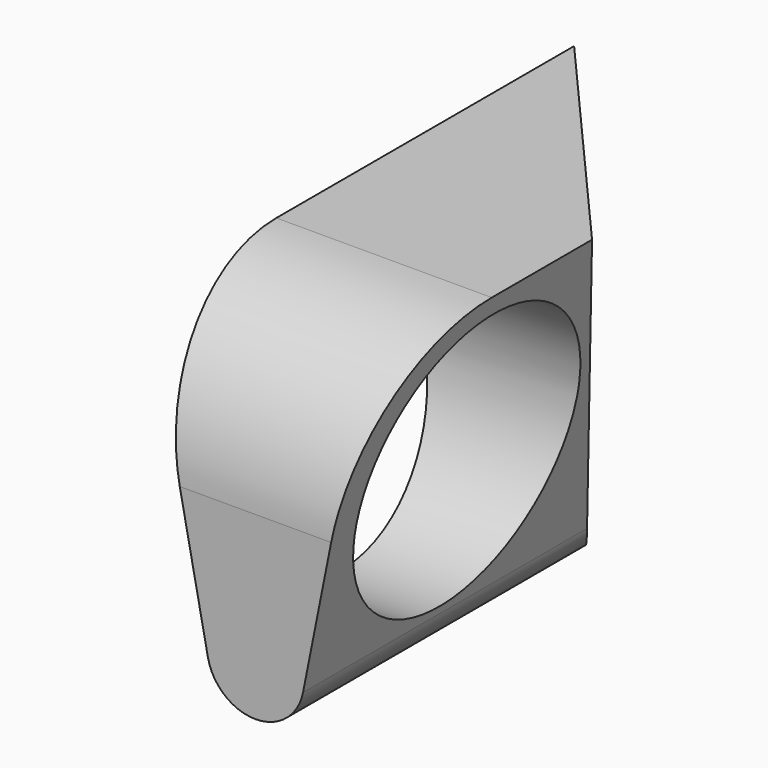
from build123d import *

# Parameters (mm, degrees)
F1_DEPTH      = 25
F2_T1_DEPTH   = 79.8532648187
F4_DEPTH      = 25
F4_DEPTH_BACK = 25
F5_T1_DEPTH   = 107.1220330496
F7_DEPTH      = 25
F8_R          = 6.2148490945
F9_DEPTH      = 25
F9_DEPTH_BACK = 25
F10_R         = 7.2426406871


# Not quite as in the source:
# - a fillet or chamfer that OpenCascade refuses, or shapes differently, is made with other operations: its cross-section is extruded or revolved along the edge and cut away or added


with BuildPart() as f1:
    # F0 (on Front) → F1 (new body)
    with BuildSketch(Plane.XZ):
        Polygon((4.8560337164, 7.4956272729), (0, 7.4956272729), (-4.8560337164, 7.4956272729), (0, -16.87037386), align=None)
    extrude(amount=F1_DEPTH)

    # F2: fillet of radius 2.1864014695 on 1 edges, made by hand

    # F2_s2 → F2_t1 (cut)
    with BuildSketch(Plane.XZ.offset(-27.4266324093)):
        with BuildLine():
            ThreePointArc((-2.1442330518, -6.1113083304), (0, -7.87037386), (2.1442330518, -6.1113083304))
            Line((2.1442330518, -6.1113083304), (0, -16.87037386))
            Line((0, -16.87037386), (-2.1442330518, -6.1113083304))
        make_face()
    extrude(amount=F2_T1_DEPTH, mode=Mode.SUBTRACT)

    # F3 (on Right) → F4 (cut, two sides)
    with BuildSketch(Plane.YZ) as f4_sk:
        with BuildLine():
            ThreePointArc((1.5301647967, 9.1992565168), (-4.4063240448, -7.9303751627), (-16.6751330548, -21.2773788233))
            Line((-16.6751330548, -21.2773788233), (1.5301647967, -21.2773788233))
            Line((1.5301647967, -21.2773788233), (1.5301647967, 9.1992565168))
        make_face()
    extrude(amount=-F4_DEPTH, mode=Mode.SUBTRACT)
    extrude(f4_sk.sketch, amount=F4_DEPTH_BACK, mode=Mode.SUBTRACT)

    # F5: chamfer of 5.5 on 1 edges, made by hand

    # F5_s2 → F5_t1 (cut)
    with BuildSketch(Plane.YZ.offset(-53.5610165248)):
        with BuildLine():
            Line((0.079428002, 10.2204041802), (-9.7965992647, -15.2892315683))
            Line((-9.7965992647, -15.2892315683), (-9.7152756624, -15.3633022893))
            ThreePointArc((-9.7152756624, -15.3633022893), (-3.8594523105, -7.2118040219), (0.1053121044, 2.0189976591))
            Line((0.1053121044, 2.0189976591), (0.11, 2.0507680961))
            ThreePointArc((0.11, 2.0507680961), (0.11, 6.1355861381), (0.189428002, 10.2204041802))
            Line((0.189428002, 10.2204041802), (0.079428002, 10.2204041802))
        make_face()
    extrude(amount=F5_T1_DEPTH, mode=Mode.SUBTRACT)

    # F6 (on face) → F7 (cut)
    with BuildSketch(Plane.XY.offset(7.4956272729)):
        Polygon((7.9051312059, 6.1967439927), (-4.8560337164, -0.9754663641), (7.9051312059, -15.5989079942), align=None)
    extrude(amount=-F7_DEPTH, mode=Mode.SUBTRACT)

    # F8 (on Right) → F9 (cut, two sides)
    with BuildSketch(Plane.YZ) as f9_sk:
        with Locations((-17.4094103277, 0.4502551164)):
            Circle(F8_R)
    extrude(amount=F9_DEPTH, mode=Mode.SUBTRACT)
    extrude(f9_sk.sketch, amount=-F9_DEPTH_BACK, mode=Mode.SUBTRACT)

    # F10
    f10_edges = [f1.edges().sort_by_distance(p)[0] for p in [
        (0, -25, 7.495627),
    ]]
    fillet(f10_edges, radius=F10_R)


solid = f1.part
